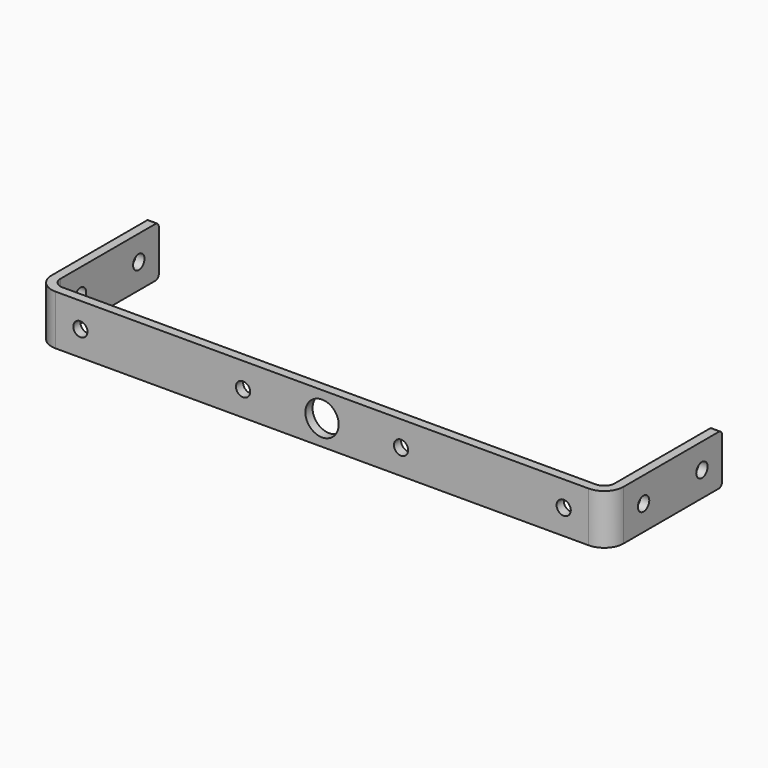
from build123d import *

# Parameters (mm, degrees)
F1_DEPTH = 9.525
F2_R     = 1.98374
F3_R     = 3.69316
F4_R     = 1.35255
F5_DEPTH = 108.98632
F6_R     = 1.35255
F6_R_2   = 3.175
F7_DEPTH = 1.70942
F8_R     = 0.762


with BuildPart() as f1:
    # F0 (on Top) → F1 (new body)
    with BuildSketch(Plane.XY):
        Polygon((0, 25.4), (0, 0), (-105.56748, 0), (-105.56748, 25.4), (-107.2769, 25.4), (-107.2769, -1.70942), (1.70942, -1.70942), (1.70942, 25.4), align=None)
    extrude(amount=F1_DEPTH)

    # F2
    f2_edges = [f1.edges().sort_by_distance(p)[0] for p in [
        (0, 0, 4.7625),
        (-105.56748, 0, 4.7625),
    ]]
    fillet(f2_edges, radius=F2_R)

    # F3
    f3_edges = [f1.edges().sort_by_distance(p)[0] for p in [
        (1.70942, -1.70942, 4.7625),
        (-107.2769, -1.70942, 4.7625),
    ]]
    fillet(f3_edges, radius=F3_R)

    # F4 (on face) → F5 (cut, through all)
    with BuildSketch(Plane(origin=(-107.2769, 0, 0), x_dir=(0, -1, 0), z_dir=(-1, 0, 0))):
        with Locations((-20.6375, 4.7625)):
            Circle(F4_R)
        with Locations((-6.74624, 4.7625)):
            Circle(F4_R)
    extrude(amount=-F5_DEPTH, mode=Mode.SUBTRACT)

    # F6 (on face) → F7 (cut, through all)
    with BuildSketch(Plane.XZ.offset(1.70942)):
        with Locations((-98.82124, 4.7625)):
            Circle(F6_R)
        with Locations((-6.74624, 4.7625)):
            Circle(F6_R)
        with Locations((-67.8351831, 4.7625)):
            Circle(F6_R)
        with Locations((-37.7322969, 4.7625)):
            Circle(F6_R)
        with Locations((-52.78374, 4.7625)):
            Circle(F6_R_2)
    extrude(amount=-F7_DEPTH, mode=Mode.SUBTRACT)

    # F8
    f8_edges = [f1.edges().sort_by_distance(p)[0] for p in [
        (-106.42219, 25.4, 9.525),
        (-106.42219, 25.4, 0),
        (0.85471, 25.4, 9.525),
        (0.85471, 25.4, 0),
    ]]
    fillet(f8_edges, radius=F8_R)


solid = f1.part
